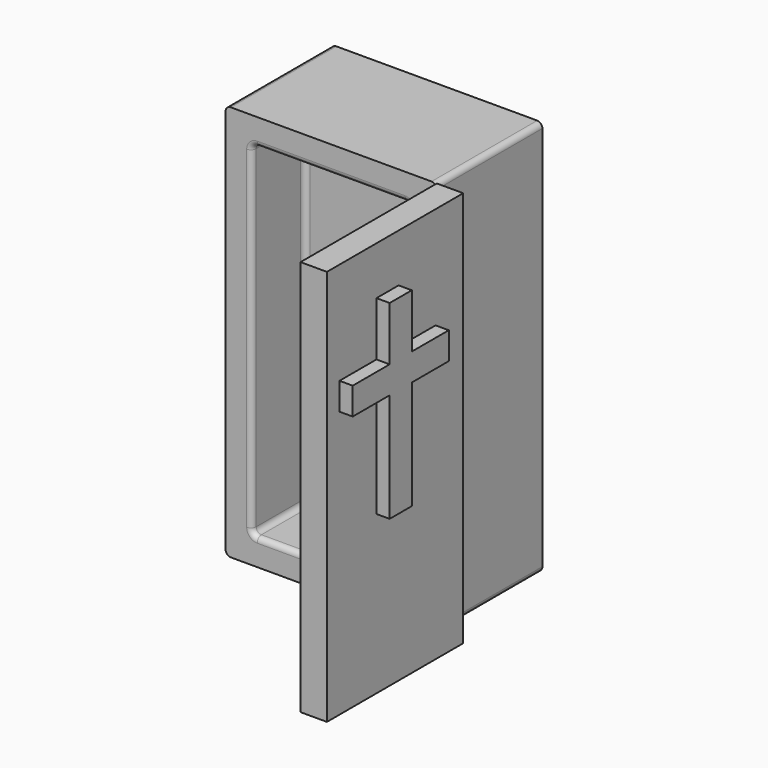
from build123d import *

# Parameters (mm, degrees)
F0_W         = 203.2
F0_H         = 381.1146762907
F1_DEPTH     = 127
F2_T         = -25.4
F3_W         = 163.8680438995
F3_H         = 381.1146762907
F4_DEPTH     = 25.4
F5_W         = 152.4
F5_H         = 330.3146762907
F6_DEPTH     = 38.1
F7_T1_DEPTH  = 320.1546762907
F7_T3_DEPTH  = 142.24
F7_T5_DEPTH  = 58.42
F7_S9_W      = 5.08
F7_S9_H      = 5.08
F7_T10_DEPTH = 5.08
F7_S15_W     = 5.08
F7_S15_H     = 5.08
F7_T16_DEPTH = 5.08
F7_S21_W     = 5.08
F7_S21_H     = 5.08
F7_T22_DEPTH = 5.08
F7_S27_W     = 5.08
F7_S27_H     = 5.08
F7_T28_DEPTH = 5.08
F7_T31_DEPTH = 152.4
F7_T33_DEPTH = 142.24
F7_T35_DEPTH = 320.1546762907
F7_T38_ANGLE = 90
F7_T40_ANGLE = 90
F7_T42_ANGLE = 90
F7_T44_ANGLE = 90
F9_DEPTH     = 12.7


# Not quite as in the source:
# - a fillet or chamfer that OpenCascade refuses, or shapes differently, is made with other operations: its cross-section is extruded or revolved along the edge and cut away or added


with BuildPart() as f1:
    # F0 (on Front) → F1 (new body)
    with BuildSketch(Plane.XZ):
        with Locations((33.975193277, -74.0627218038)):
            Rectangle(F0_W, F0_H)
    extrude(amount=F1_DEPTH)

    # F2
    f2_openings = [f1.faces().sort_by_distance(p)[0] for p in [
        (33.975193, -127, -74.062722),
    ]]
    offset(amount=F2_T, openings=f2_openings)

    # F3 (on face) → F4 (join)
    with BuildSketch(Plane.YZ.offset(135.575193277)):
        with Locations((-208.9340219498, -74.0627218038)):
            Rectangle(F3_W, F3_H)
    extrude(amount=F4_DEPTH)

    # F5 (on face) → F6 (join)
    with BuildSketch(Plane.XZ.offset(25.4)):
        with Locations((33.975193277, -74.0627218038)):
            Rectangle(F5_W, F5_H)
    extrude(amount=F6_DEPTH)

    # F7: fillet of radius 5.08 on 16 edges, made by hand

    # F7_s2 → F7_t1 (join)
    with BuildSketch(Plane.XY.offset(-234.1400599492)):
        with BuildLine():
            ThreePointArc((-42.224806723, -68.58), (-40.7369091714, -64.9878975516), (-37.144806723, -63.5))
            Line((-37.144806723, -63.5), (-42.224806723, -63.5))
            Line((-42.224806723, -63.5), (-42.224806723, -68.58))
        make_face()
        with BuildLine():
            ThreePointArc((110.175193277, -68.58), (108.6872957254, -64.9878975516), (105.095193277, -63.5))
            Line((105.095193277, -63.5), (110.175193277, -63.5))
            Line((110.175193277, -63.5), (110.175193277, -68.58))
        make_face()
    extrude(amount=F7_T1_DEPTH)

    # F7_s4 → F7_t3 (join)
    with BuildSketch(Plane.YZ.offset(-37.144806723)):
        with BuildLine():
            ThreePointArc((-68.58, 91.0946163416), (-64.9878975516, 89.60671879), (-63.5, 86.0146163416))
            Line((-63.5, 86.0146163416), (-63.5, 91.0946163416))
            Line((-63.5, 91.0946163416), (-68.58, 91.0946163416))
        make_face()
        with BuildLine():
            ThreePointArc((-68.58, -239.2200599492), (-64.9878975516, -237.7321623976), (-63.5, -234.1400599492))
            Line((-63.5, -234.1400599492), (-63.5, -239.2200599492))
            Line((-63.5, -239.2200599492), (-68.58, -239.2200599492))
        make_face()
    extrude(amount=F7_T3_DEPTH)

    # F7_s6 → F7_t5 (join)
    with BuildSketch(Plane.XZ.offset(68.58)):
        with BuildLine():
            ThreePointArc((-42.224806723, 86.0146163416), (-40.7369091714, 89.60671879), (-37.144806723, 91.0946163416))
            Line((-37.144806723, 91.0946163416), (-42.224806723, 91.0946163416))
            Line((-42.224806723, 91.0946163416), (-42.224806723, 86.0146163416))
        make_face()
        with BuildLine():
            ThreePointArc((110.175193277, 86.0146163416), (108.6872957254, 89.60671879), (105.095193277, 91.0946163416))
            Line((105.095193277, 91.0946163416), (110.175193277, 91.0946163416))
            Line((110.175193277, 91.0946163416), (110.175193277, 86.0146163416))
        make_face()
        with BuildLine():
            ThreePointArc((110.175193277, -234.1400599492), (108.6872957254, -237.7321623976), (105.095193277, -239.2200599492))
            Line((105.095193277, -239.2200599492), (110.175193277, -239.2200599492))
            Line((110.175193277, -239.2200599492), (110.175193277, -234.1400599492))
        make_face()
        with BuildLine():
            ThreePointArc((-37.144806723, -239.2200599492), (-40.7369091714, -237.7321623976), (-42.224806723, -234.1400599492))
            Line((-42.224806723, -234.1400599492), (-42.224806723, -239.2200599492))
            Line((-42.224806723, -239.2200599492), (-37.144806723, -239.2200599492))
        make_face()
    extrude(amount=F7_T5_DEPTH)


with BuildPart() as f7_tool8:
    # F7_s9 → F7_t10 (new body)
    with BuildSketch(Plane.YZ.offset(-37.144806723)):
        with Locations((-66.04, 88.5546163416)):
            Rectangle(F7_S9_W, F7_S9_H)
    extrude(amount=-F7_T10_DEPTH)

    # F7_s11 → F7_t12 (revolve, cut)
    with BuildSketch(Plane(origin=(-37.144806723, -68.58, 86.0146163416), x_dir=(0, -0.7071067812, -0.7071067812), z_dir=(0, 0.7071067812, -0.7071067812))):
        with BuildLine():
            ThreePointArc((0, -5.08), (5.08, 0), (0, 5.08))
            Line((0, 5.08), (0, -5.08))
        make_face()
    revolve(axis=Axis((-37.144806723, -68.58, 86.0146163416), (-1, 0, 0)), mode=Mode.SUBTRACT)


with BuildPart() as f1_1:
    add(f1.part)

    # F7_t7: union F7_tool8
    add(f7_tool8.part)


with BuildPart() as f7_tool14:
    # F7_s15 → F7_t16 (new body)
    with BuildSketch(Plane.YZ.offset(-37.144806723)):
        with Locations((-66.04, -236.6800599492)):
            Rectangle(F7_S15_W, F7_S15_H)
    extrude(amount=-F7_T16_DEPTH)

    # F7_s17 → F7_t18 (revolve, cut)
    with BuildSketch(Plane(origin=(-37.144806723, -68.58, -234.1400599492), x_dir=(0, -0.7071067812, 0.7071067812), z_dir=(0, -0.7071067812, -0.7071067812))):
        with BuildLine():
            ThreePointArc((0, -5.08), (5.08, 0), (0, 5.08))
            Line((0, 5.08), (0, -5.08))
        make_face()
    revolve(axis=Axis((-37.144806723, -68.58, -234.1400599492), (-1, 0, 0)), mode=Mode.SUBTRACT)


with BuildPart() as f1_2:
    add(f1_1.part)

    # F7_t13: union F7_tool14
    add(f7_tool14.part)


with BuildPart() as f7_tool20:
    # F7_s21 → F7_t22 (new body)
    with BuildSketch(Plane.XY.offset(86.0146163416)):
        with Locations((107.635193277, -66.04)):
            Rectangle(F7_S21_W, F7_S21_H)
    extrude(amount=F7_T22_DEPTH)

    # F7_s23 → F7_t24 (revolve, cut)
    with BuildSketch(Plane(origin=(105.095193277, -68.58, 86.0146163416), x_dir=(-0.7071067812, -0.7071067812, 0), z_dir=(-0.7071067812, 0.7071067812, 0))):
        with BuildLine():
            ThreePointArc((0, -5.08), (5.08, 0), (0, 5.08))
            Line((0, 5.08), (0, -5.08))
        make_face()
    revolve(axis=Axis((105.095193277, -68.58, 86.0146163416), (0, 0, 1)), mode=Mode.SUBTRACT)


with BuildPart() as f1_3:
    add(f1_2.part)

    # F7_t19: union F7_tool20
    add(f7_tool20.part)


with BuildPart() as f7_tool26:
    # F7_s27 → F7_t28 (new body)
    with BuildSketch(Plane.XZ.offset(68.58)):
        with Locations((107.635193277, -236.6800599492)):
            Rectangle(F7_S27_W, F7_S27_H)
    extrude(amount=-F7_T28_DEPTH)

    # F7_s29 → F7_t30 (revolve, cut)
    with BuildSketch(Plane(origin=(105.095193277, -68.58, -234.1400599492), x_dir=(-0.7071067812, 0, 0.7071067812), z_dir=(-0.7071067812, 0, -0.7071067812))):
        with BuildLine():
            ThreePointArc((0, -5.08), (5.08, 0), (0, 5.08))
            Line((0, 5.08), (0, -5.08))
        make_face()
    revolve(axis=Axis((105.095193277, -68.58, -234.1400599492), (0, 1, 0)), mode=Mode.SUBTRACT)


with BuildPart() as f1_4:
    add(f1_3.part)

    # F7_t25: union F7_tool26
    add(f7_tool26.part)

    # F7_s32 → F7_t31 (cut)
    with BuildSketch(Plane.XZ.offset(-12.7)):
        with BuildLine():
            ThreePointArc((-62.544806723, -264.6200599492), (-66.1369091714, -263.1321623976), (-67.624806723, -259.5400599492))
            Line((-67.624806723, -259.5400599492), (-67.624806723, -264.6200599492))
            Line((-67.624806723, -264.6200599492), (-62.544806723, -264.6200599492))
        make_face()
        with BuildLine():
            ThreePointArc((135.575193277, -259.5400599492), (134.0872957254, -263.1321623976), (130.495193277, -264.6200599492))
            Line((130.495193277, -264.6200599492), (135.575193277, -264.6200599492))
            Line((135.575193277, -264.6200599492), (135.575193277, -259.5400599492))
        make_face()
        with BuildLine():
            ThreePointArc((135.575193277, 111.4146163416), (134.0872957254, 115.00671879), (130.495193277, 116.4946163416))
            Line((130.495193277, 116.4946163416), (135.575193277, 116.4946163416))
            Line((135.575193277, 116.4946163416), (135.575193277, 111.4146163416))
        make_face()
        with BuildLine():
            ThreePointArc((-62.544806723, 116.4946163416), (-66.1369091714, 115.00671879), (-67.624806723, 111.4146163416))
            Line((-67.624806723, 111.4146163416), (-67.624806723, 116.4946163416))
            Line((-67.624806723, 116.4946163416), (-62.544806723, 116.4946163416))
        make_face()
    extrude(amount=F7_T31_DEPTH, mode=Mode.SUBTRACT)

    # F7_s34 → F7_t33 (cut)
    with BuildSketch(Plane.YZ.offset(-37.144806723)):
        with BuildLine():
            ThreePointArc((-127, 96.1746163416), (-125.5121024484, 92.5825138932), (-121.92, 91.0946163416))
            Line((-121.92, 91.0946163416), (-127, 91.0946163416))
            Line((-127, 91.0946163416), (-127, 96.1746163416))
        make_face()
        with BuildLine():
            ThreePointArc((-127, -244.3000599492), (-125.5121024484, -240.7079575007), (-121.92, -239.2200599492))
            Line((-121.92, -239.2200599492), (-127, -239.2200599492))
            Line((-127, -239.2200599492), (-127, -244.3000599492))
        make_face()
    extrude(amount=F7_T33_DEPTH, mode=Mode.SUBTRACT)

    # F7_s36 → F7_t35 (cut)
    with BuildSketch(Plane.XY.offset(-234.1400599492)):
        with BuildLine():
            ThreePointArc((115.255193277, -127), (111.6630908286, -125.5121024484), (110.175193277, -121.92))
            Line((110.175193277, -121.92), (110.175193277, -127))
            Line((110.175193277, -127), (115.255193277, -127))
        make_face()
        with BuildLine():
            ThreePointArc((-47.304806723, -127), (-43.7127042746, -125.5121024484), (-42.224806723, -121.92))
            Line((-42.224806723, -121.92), (-42.224806723, -127))
            Line((-42.224806723, -127), (-47.304806723, -127))
        make_face()
    extrude(amount=F7_T35_DEPTH, mode=Mode.SUBTRACT)

    # F7_s37 → F7_t38 (revolve, cut)
    with BuildSketch(Plane.XY.offset(86.0146163416)):
        with BuildLine():
            ThreePointArc((-47.304806723, -127), (-43.7127042746, -125.5121024484), (-42.224806723, -121.92))
            Line((-42.224806723, -121.92), (-42.224806723, -127))
            Line((-42.224806723, -127), (-47.304806723, -127))
        make_face()
    revolve(axis=Axis((-37.144806723, -127, 86.0146163416), (0, 1, 0)), revolution_arc=F7_T38_ANGLE, mode=Mode.SUBTRACT)

    # F7_s39 → F7_t40 (revolve, cut)
    with BuildSketch(Plane.YZ.offset(-37.144806723)):
        with BuildLine():
            ThreePointArc((-127, -244.3000599492), (-125.5121024484, -240.7079575007), (-121.92, -239.2200599492))
            Line((-121.92, -239.2200599492), (-127, -239.2200599492))
            Line((-127, -239.2200599492), (-127, -244.3000599492))
        make_face()
    revolve(axis=Axis((-37.144806723, -127, -234.1400599492), (0, 1, 0)), revolution_arc=F7_T40_ANGLE, mode=Mode.SUBTRACT)

    # F7_s41 → F7_t42 (revolve, cut)
    with BuildSketch(Plane.XY.offset(-234.1400599492)):
        with BuildLine():
            ThreePointArc((115.255193277, -127), (111.6630908286, -125.5121024484), (110.175193277, -121.92))
            Line((110.175193277, -121.92), (110.175193277, -127))
            Line((110.175193277, -127), (115.255193277, -127))
        make_face()
    revolve(axis=Axis((105.095193277, -127, -234.1400599492), (0, 1, 0)), revolution_arc=F7_T42_ANGLE, mode=Mode.SUBTRACT)

    # F7_s43 → F7_t44 (revolve, cut)
    with BuildSketch(Plane.XY.offset(86.0146163416)):
        with BuildLine():
            ThreePointArc((115.255193277, -127), (111.6630908286, -125.5121024484), (110.175193277, -121.92))
            Line((110.175193277, -121.92), (110.175193277, -127))
            Line((110.175193277, -127), (115.255193277, -127))
        make_face()
    revolve(axis=Axis((105.095193277, -127, 86.0146163416), (0, -1, 0)), revolution_arc=F7_T44_ANGLE, mode=Mode.SUBTRACT)


with BuildPart() as f9:
    # F8 (on face) → F9 (new body)
    with BuildSketch(Plane.YZ.offset(160.975193277)):
        Polygon((-204.7111040329, 70.0232706935), (-231.2980165388, 70.0232706935), (-231.2980165388, 18.0956996665), (-275.7480165388, 18.0956996665), (-275.7480165388, -8.0757932739), (-231.2980165388, -8.0757932739), (-231.2980165388, -112.7617754013), (-204.7111040329, -112.7617754013), (-204.7111040329, -8.0757932739), (-160.2611040329, -8.0757932739), (-160.2611040329, 18.0956996665), (-204.7111040329, 18.0956996665), align=None)
    extrude(amount=F9_DEPTH)


solid = Compound([f1_4.part, f9.part])
